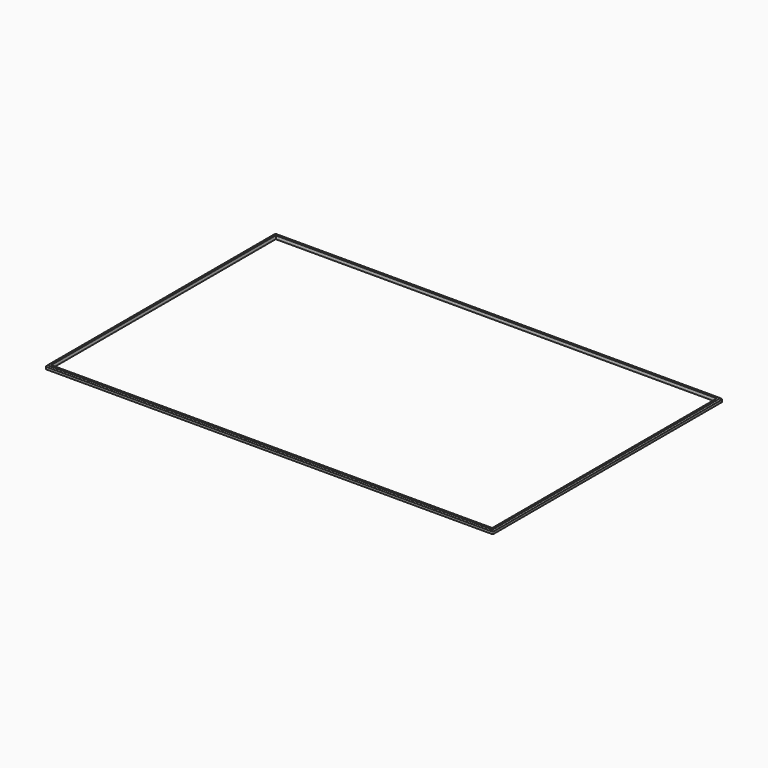
from build123d import *

# Parameters (mm, degrees)
F0_W     = 399
F0_H     = 256
F0_W_2   = 393.4
F0_H_2   = 250.4
F1_DEPTH = 1.5
F2_SIZE  = 1
F3_F1_R  = 1
F3_F2_R  = 1
F3_F3_R  = 1
F3_F4_R  = 1
F3_F5_R  = 1
F3_F6_R  = 1
F3_F7_R  = 1
F3_F8_R  = 1


with BuildPart() as f1:
    # F0 (on Top) → F1 (new body, symmetric)
    with BuildSketch(Plane.XY):
        Rectangle(F0_W, F0_H)
        Rectangle(F0_W_2, F0_H_2, mode=Mode.SUBTRACT)
    extrude(amount=F1_DEPTH, both=True)

    # F2
    f2_edges = [f1.edges().sort_by_distance(p)[0] for p in [
        (0, -128, 1.5),
        (-199.5, 0, 1.5),
        (0, 128, 1.5),
        (199.5, 0, 1.5),
    ]]
    chamfer(f2_edges, length=F2_SIZE)

    # F3: fillet of radius 1 on 8 edges, made by hand

    # F3_f1
    f3_f1_edges = [f1.edges().sort_by_distance(p)[0] for p in [
        (199.5, 128, -0.5),
    ]]
    fillet(f3_f1_edges, radius=F3_F1_R)

    # F3_f2
    f3_f2_edges = [f1.edges().sort_by_distance(p)[0] for p in [
        (199.5, -128, -0.5),
    ]]
    fillet(f3_f2_edges, radius=F3_F2_R)

    # F3_f3
    f3_f3_edges = [f1.edges().sort_by_distance(p)[0] for p in [
        (-199.5, 128, -0.5),
    ]]
    fillet(f3_f3_edges, radius=F3_F3_R)

    # F3_f4
    f3_f4_edges = [f1.edges().sort_by_distance(p)[0] for p in [
        (198.8535533906, -127.3535533906, 1.1464466094),
    ]]
    fillet(f3_f4_edges, radius=F3_F4_R)

    # F3_f5
    f3_f5_edges = [f1.edges().sort_by_distance(p)[0] for p in [
        (198.8535533906, 127.3535533906, 1.1464466094),
    ]]
    fillet(f3_f5_edges, radius=F3_F5_R)

    # F3_f6
    f3_f6_edges = [f1.edges().sort_by_distance(p)[0] for p in [
        (-199.5, -128, -0.5),
    ]]
    fillet(f3_f6_edges, radius=F3_F6_R)

    # F3_f7
    f3_f7_edges = [f1.edges().sort_by_distance(p)[0] for p in [
        (-198.8535533906, 127.3535533906, 1.1464466094),
    ]]
    fillet(f3_f7_edges, radius=F3_F7_R)

    # F3_f8
    f3_f8_edges = [f1.edges().sort_by_distance(p)[0] for p in [
        (-198.8535533906, -127.3535533906, 1.1464466094),
    ]]
    fillet(f3_f8_edges, radius=F3_F8_R)


solid = f1.part
